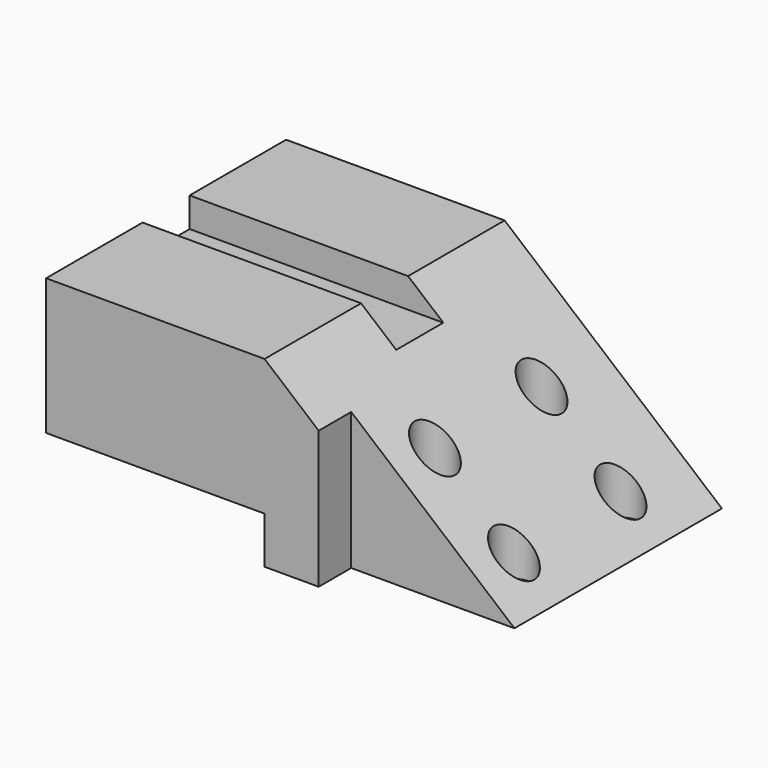
from build123d import *

# Parameters (mm, degrees)
F1_DEPTH = 76.2
F2_W     = 14.9392048001
F2_H     = 7.519736886
F3_DEPTH = 110.691522939
F4_W     = 41.4504492655
F4_H     = 10.3266900301
F4_R     = 5.148684062
F5_DEPTH = 188


# Not quite as in the source:
# - an extrude ends at something that could not be found from the text; its depth is read off the source's solid


with BuildPart() as f1:
    # F0 (on Front) → F1 (new body)
    with BuildSketch(Plane.XZ):
        Polygon((0, 11.8811847642), (0, 0), (55.1948659122, 0), (0, 46.4719720185), (-55.4956570268, 46.4719720185), (-55.4956570268, 11.8811847642), align=None)
    extrude(amount=F1_DEPTH)

    # F2 (on face) → F3 (cut, through all)
    with BuildSketch(Plane(origin=(-55.4956570268, 0, 0), x_dir=(0, -1, 0), z_dir=(-1, 0, 0))):
        with Locations((38.1, 42.7121035755)):
            Rectangle(F2_W, F2_H)
    extrude(amount=-F3_DEPTH, mode=Mode.SUBTRACT)

    # F4 (on Top) → F5 (cut, through all)
    with BuildSketch(Plane.XY):
        with Locations((34.4696412794, -71.036654985)):
            Rectangle(F4_W, F4_H)
        with Locations((45.0900119481, -53.3901341259)):
            Circle(F4_R)
        with Locations((45.0900119481, -19.5571203102)):
            Circle(F4_R)
        with Locations((25.0240119481, -53.3901341259)):
            Circle(F4_R)
        with Locations((25.0240119481, -19.5571203102)):
            Circle(F4_R)
    extrude(amount=F5_DEPTH, mode=Mode.SUBTRACT)


solid = f1.part
